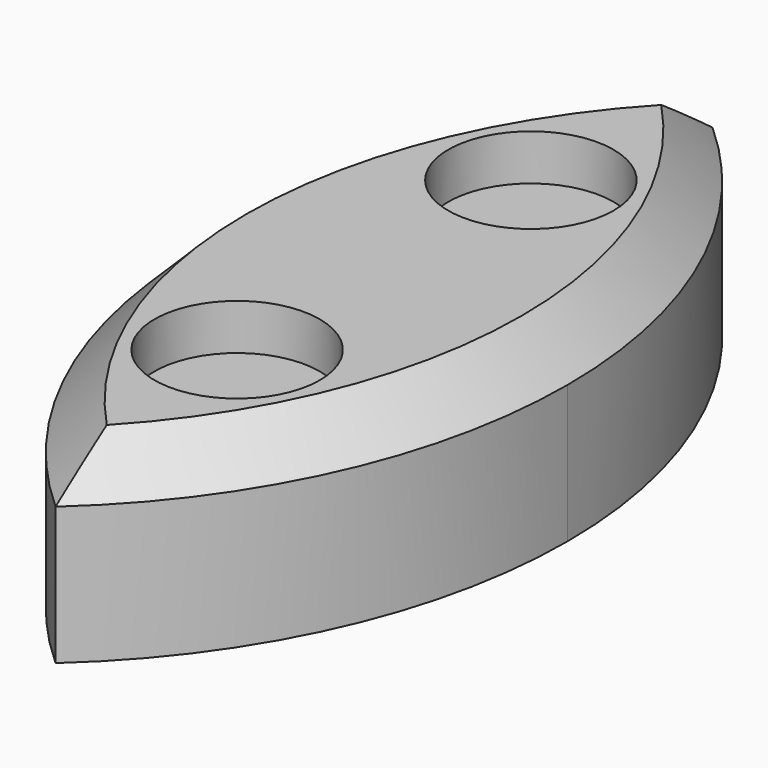
from build123d import *

# Parameters (mm, degrees)
F0_R        = 9
F1_DEPTH    = 20
F2_DEPTH    = 15
F3_T2_ANGLE = 120.9484473771
F3_T4_ANGLE = 120.9484473771


# Not quite as in the source:
# - a fillet or chamfer that OpenCascade refuses, or shapes differently, is made with other operations: its cross-section is extruded or revolved along the edge and cut away or added


with BuildPart() as f1:
    # F0 (on Top) → F1 (new body)
    with BuildSketch(Plane.XY):
        with BuildLine():
            Line((-20, 0), (0, 0))
            Line((0, 0), (20, 0))
            ThreePointArc((20, 0), (14.7722557505, 24.4948974278), (0, 44.72135955))
            ThreePointArc((0, 44.72135955), (-14.7722557505, 24.4948974278), (-20, 0))
        make_face()
        with Locations((0, 20)):
            Circle(F0_R, mode=Mode.SUBTRACT)
        with BuildLine():
            Line((20, 0), (0, 0))
            Line((0, 0), (-20, 0))
            ThreePointArc((-20, 0), (-14.7722557505, -24.4948974278), (0, -44.72135955))
            ThreePointArc((0, -44.72135955), (14.7722557505, -24.4948974278), (20, 0))
        make_face()
        with Locations((0, -20)):
            Circle(F0_R, mode=Mode.SUBTRACT)
    extrude(amount=F1_DEPTH)

    # F0 (on Top) → F2 (join)
    with BuildSketch(Plane.XY):
        with Locations((0, -20)):
            Circle(F0_R)
        with Locations((0, 20)):
            Circle(F0_R)
    extrude(amount=F2_DEPTH)

    # F3: chamfer of 5 on 2 edges, made by hand

    # F3_s1 → F3_t2 (revolve, cut)
    with BuildSketch(Plane(origin=(-30.2853323821, -17.1526073175, 0), x_dir=(0, 0, 1), z_dir=(-0.8701340756, -0.4928150672, 0))):
        Polygon((15, -40.2873973125), (20, -35.2873973125), (20, -40.2873973125), align=None)
    revolve(axis=Axis((-40, 0, 20), (0, 0, 1)), revolution_arc=F3_T2_ANGLE, mode=Mode.SUBTRACT)

    # F3_s3 → F3_t4 (revolve, cut)
    with BuildSketch(Plane(origin=(30.2853323821, 17.1526073175, 0), x_dir=(0, 0, 1), z_dir=(0.8701340756, 0.4928150672, 0))):
        Polygon((15, -40.2873973125), (20, -35.2873973125), (20, -40.2873973125), align=None)
    revolve(axis=Axis((40, 0, 20), (0, 0, 1)), revolution_arc=F3_T4_ANGLE, mode=Mode.SUBTRACT)


solid = f1.part
